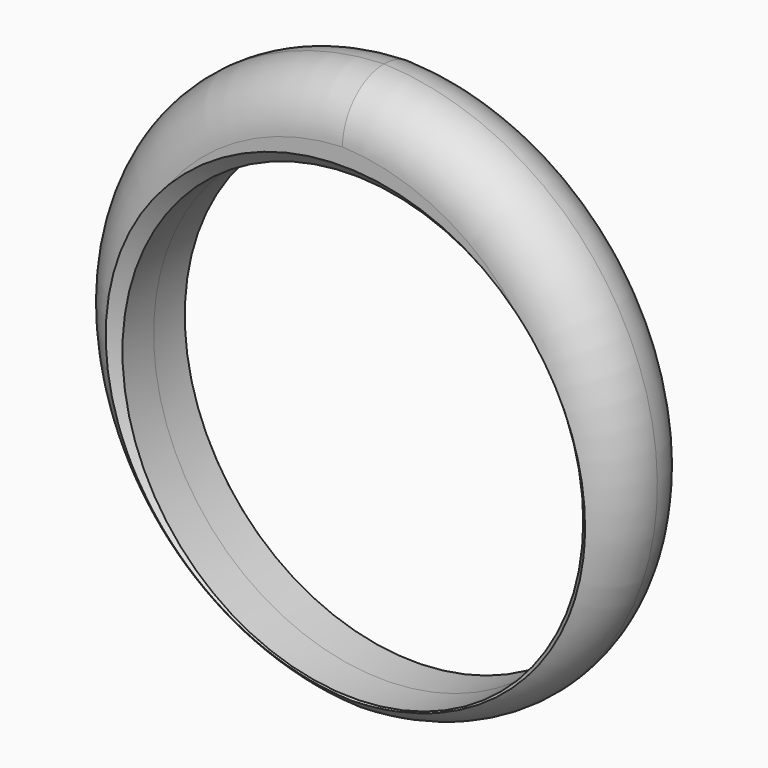
from build123d import *

# Parameters (mm, degrees)
F0_R          = 8.875
F1_DEPTH      = 2
F1_DEPTH_BACK = 2
F2_SIZE       = 0.5
F3_T2_ANGLE   = 229.39221369
F3_T4_ANGLE   = 229.39221369
F3_T6_ANGLE   = 229.39221369
F3_T8_ANGLE   = 229.39221369


# Not quite as in the source:
# - a fillet or chamfer that OpenCascade refuses, or shapes differently, is made with other operations: its cross-section is extruded or revolved along the edge and cut away or added


with BuildPart() as f1:
    # F0 (on Front) → F1 (new body, two sides)
    with BuildSketch(Plane.XZ) as f1_sk:
        with BuildLine():
            ThreePointArc((9.0113523195, 6.7058048682), (5.1879898372, 10.5200364151), (0, 12.0204444975))
            ThreePointArc((0, 12.0204444975), (-5.1879898372, 10.5200364151), (-9.0113523195, 6.7058048682))
            ThreePointArc((-9.0113523195, 6.7058048682), (-9.186793263, -4.0631742687), (0, -9.6849640831))
            ThreePointArc((0, -9.6849640831), (9.186793263, -4.0631742687), (9.0113523195, 6.7058048682))
        make_face()
        Circle(F0_R, mode=Mode.SUBTRACT)
    extrude(amount=F1_DEPTH)
    extrude(f1_sk.sketch, amount=-F1_DEPTH_BACK)

    # F2
    f2_edges = [f1.edges().sort_by_distance(p)[0] for p in [
        (-8.875, 2, 0),
        (-8.875, -2, 0),
    ]]
    chamfer(f2_edges, length=F2_SIZE)

    # F3: fillet of radius 2 on 4 edges, made by hand

    # F3_s1 → F3_t2 (revolve, cut)
    with BuildSketch(Plane(origin=(-0.7137842207, 0, 0.3282453014), x_dir=(0, 1, 0), z_dir=(-0.9085365688, 0, 0.4178053412))):
        with BuildLine():
            ThreePointArc((2, 7.9336436901), (1.4142135624, 9.3478572525), (0, 9.9336436901))
            Line((0, 9.9336436901), (2, 9.9336436901))
            Line((2, 9.9336436901), (2, 7.9336436901))
        make_face()
    revolve(axis=Axis((-0.3277288129, 2, 1.1677402072), (0, -1, 0)), revolution_arc=F3_T2_ANGLE, mode=Mode.SUBTRACT)

    # F3_s3 → F3_t4 (revolve, cut)
    with BuildSketch(Plane(origin=(-0.1727441321, 0, 0.0794392031), x_dir=(0, 1, 0), z_dir=(0.9085365688, 0, -0.4178053412))):
        with BuildLine():
            ThreePointArc((2, 10.0555130523), (1.4142135624, 11.4697266146), (0, 12.0555130523))
            Line((0, 12.0555130523), (2, 12.0555130523))
            Line((2, 12.0555130523), (2, 10.0555130523))
        make_face()
    revolve(axis=Axis((0.3277288129, 2, 1.1677402072), (0, -1, 0)), revolution_arc=F3_T4_ANGLE, mode=Mode.SUBTRACT)

    # F3_s5 → F3_t6 (revolve, cut)
    with BuildSketch(Plane(origin=(0.1727441321, 0, 0.0794392031), x_dir=(0, 1, 0), z_dir=(-0.9085365688, 0, -0.4178053412))):
        with BuildLine():
            ThreePointArc((0, -12.0555130523), (-1.4142135624, -11.4697266146), (-2, -10.0555130523))
            Line((-2, -10.0555130523), (-2, -12.0555130523))
            Line((-2, -12.0555130523), (0, -12.0555130523))
        make_face()
    revolve(axis=Axis((-0.3277288129, -2, 1.1677402072), (0, 1, 0)), revolution_arc=F3_T6_ANGLE, mode=Mode.SUBTRACT)

    # F3_s7 → F3_t8 (revolve, cut)
    with BuildSketch(Plane(origin=(0.7137842207, 0, 0.3282453014), x_dir=(0, 1, 0), z_dir=(0.9085365688, 0, 0.4178053412))):
        with BuildLine():
            ThreePointArc((0, -9.9336436901), (-1.4142135624, -9.3478572525), (-2, -7.9336436901))
            Line((-2, -7.9336436901), (-2, -9.9336436901))
            Line((-2, -9.9336436901), (0, -9.9336436901))
        make_face()
    revolve(axis=Axis((0.3277288129, -2, 1.1677402072), (0, 1, 0)), revolution_arc=F3_T8_ANGLE, mode=Mode.SUBTRACT)


solid = f1.part
